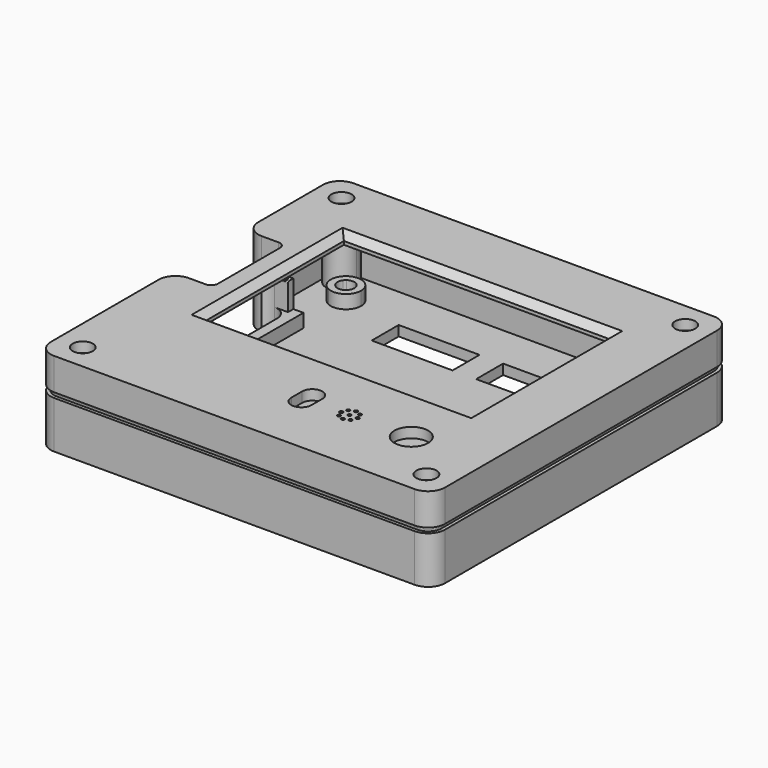
from build123d import *

# Parameters (mm, degrees)
F0_R        = 2.5
F1_DEPTH    = 15
F2_DEPTH    = 7
F0_W        = 24
F0_H        = 10
F3_DEPTH    = 3
F4_R        = 4
F5_DEPTH    = 14
F6_T1_DEPTH = 14
F7_T1_DEPTH = 14
F9_W        = 7
F9_H        = 1
F10_DEPTH   = 8
F9_R        = 0.5
F9_R_2      = 5
F9_W_2      = 79
F9_H_2      = 52
F11_DEPTH   = 3
F12_SIZE    = 2
F13_DEPTH   = 9.5
F14_R       = 0.5
F15_R       = 0.5
F9_R_3      = 1.75
F16_DEPTH   = 8
F17_R       = 3
F18_DEPTH   = 3
F19_R       = 2
F20_W       = 33
F20_H       = 2
F21_DEPTH   = 1


# Not quite as in the source:
# - a fillet or chamfer that OpenCascade refuses, or shapes differently, is made with other operations: its cross-section is extruded or revolved along the edge and cut away or added
# - a feature names something its author has since deleted; it is built from what else it names


with BuildPart() as f1:
    # F0 (on Top) → F1 (new body)
    with BuildSketch(Plane.XY):
        with BuildLine():
            Line((-46.5, 22.5), (-46.5, 24.5))
            Line((-46.5, 24.5), (-50.5, 24.5))
            ThreePointArc((-50.5, 24.5), (-54.0355339059, 25.9644660941), (-55.5, 29.5))
            Line((-55.5, 29.5), (-55.5, 48))
            ThreePointArc((-55.5, 48), (-54.1819805153, 51.1819805153), (-51, 52.5))
            Line((-51, 52.5), (51, 52.5))
            ThreePointArc((51, 52.5), (54.1819805153, 51.1819805153), (55.5, 48))
            Line((55.5, 48), (55.5, -48))
            ThreePointArc((55.5, -48), (54.1819805153, -51.1819805153), (51, -52.5))
            Line((51, -52.5), (-51, -52.5))
            ThreePointArc((-51, -52.5), (-54.1819805153, -51.1819805153), (-55.5, -48))
            Line((-55.5, -48), (-55.5, -13.5))
            ThreePointArc((-55.5, -13.5), (-54.0355339059, -9.9644660941), (-50.5, -8.5))
            Line((-50.5, -8.5), (-46.5, -8.5))
            Line((-46.5, -8.5), (-46.5, -6.5))
            Line((-46.5, -6.5), (-53.5, -6.5))
            ThreePointArc((-53.5, -6.5), (-56.3284271247, -7.6715728753), (-57.5, -10.5))
            Line((-57.5, -10.5), (-57.5, -50.5))
            ThreePointArc((-57.5, -50.5), (-56.3284271247, -53.3284271247), (-53.5, -54.5))
            Line((-53.5, -54.5), (53.5, -54.5))
            ThreePointArc((53.5, -54.5), (56.3284271247, -53.3284271247), (57.5, -50.5))
            Line((57.5, -50.5), (57.5, 50.5))
            ThreePointArc((57.5, 50.5), (56.3284271247, 53.3284271247), (53.5, 54.5))
            Line((53.5, 54.5), (-53.5, 54.5))
            ThreePointArc((-53.5, 54.5), (-56.3284271247, 53.3284271247), (-57.5, 50.5))
            Line((-57.5, 50.5), (-57.5, 26.5))
            ThreePointArc((-57.5, 26.5), (-56.3284271247, 23.6715728753), (-53.5, 22.5))
            Line((-53.5, 22.5), (-46.5, 22.5))
        make_face()
        with BuildLine():
            ThreePointArc((-51, 52.5), (-54.1819805153, 51.1819805153), (-55.5, 48))
            ThreePointArc((-55.5, 48), (-51, 43.5), (-46.5, 48))
            ThreePointArc((-46.5, 48), (-47.8180194847, 51.1819805153), (-51, 52.5))
        make_face()
        with Locations((-51, 48)):
            Circle(F0_R, mode=Mode.SUBTRACT)
        with BuildLine():
            ThreePointArc((55.5, 48), (54.1819805153, 51.1819805153), (51, 52.5))
            ThreePointArc((51, 52.5), (47.8180194847, 44.8180194847), (55.5, 48))
        make_face()
        with Locations((51, 48)):
            Circle(F0_R, mode=Mode.SUBTRACT)
        with BuildLine():
            ThreePointArc((51, -52.5), (54.1819805153, -51.1819805153), (55.5, -48))
            ThreePointArc((55.5, -48), (47.8180194847, -44.8180194847), (51, -52.5))
        make_face()
        with Locations((51, -48)):
            Circle(F0_R, mode=Mode.SUBTRACT)
        with BuildLine():
            ThreePointArc((-46.5, -48), (-51, -43.5), (-55.5, -48))
            ThreePointArc((-55.5, -48), (-54.1819805153, -51.1819805153), (-51, -52.5))
            ThreePointArc((-51, -52.5), (-47.8180194847, -51.1819805153), (-46.5, -48))
        make_face()
        with Locations((-51, -48)):
            Circle(F0_R, mode=Mode.SUBTRACT)
    extrude(amount=F1_DEPTH)

    # F0 (on Top) → F2, piece 5 (join)
    with BuildSketch(Plane.XY):
        Polygon((-43.5, 24.5), (-46.5, 24.5), (-46.5, 22.5), (-46.5, 21.5), (-46.5, -5.5), (-46.5, -6.5), (-46.5, -8.5), (-43.5, -8.5), align=None)
    extrude(amount=F2_DEPTH)



with BuildPart() as f2:
    # F0 (on Top) → F2 (new body)
    with BuildSketch(Plane.XY):
        with BuildLine():
            Line((-46.5, 43), (-46.5, 43.5))
            Line((-46.5, 43.5), (-46, 43.5))
            ThreePointArc((-46, 43.5), (-44.5, 44), (-43, 43.5))
            Line((-43, 43.5), (-40.4688711259, 43.5))
            ThreePointArc((-40.4688711259, 43.5), (-47.6819805153, 44.6819805153), (-46.5, 37.4688711259))
            Line((-46.5, 37.4688711259), (-46.5, 40))
            ThreePointArc((-46.5, 40), (-47, 41.5), (-46.5, 43))
        make_face()
        with BuildLine():
            Line((-40.4688711259, 43.5), (-43, 43.5))
            ThreePointArc((-43, 43.5), (-42.2639320225, 42.6180339887), (-42, 41.5))
            ThreePointArc((-42, 41.5), (-43.709430585, 39.1282917549), (-46.5, 40))
            Line((-46.5, 40), (-46.5, 37.4688711259))
            ThreePointArc((-46.5, 37.4688711259), (-42.1282917549, 37.6757353648), (-40, 41.5))
            ThreePointArc((-40, 41.5), (-40.1187855603, 42.5271124735), (-40.4688711259, 43.5))
        make_face()
        with BuildLine():
            Line((-46, 43.5), (-46.5, 43.5))
            Line((-46.5, 43.5), (-46.5, 43))
            ThreePointArc((-46.5, 43), (-46.267766953, 43.267766953), (-46, 43.5))
        make_face()
    extrude(amount=F2_DEPTH)


with BuildPart() as f2b:
    # F0 (on Top) → F2, piece 2 (new body)
    with BuildSketch(Plane.XY):
        with BuildLine():
            ThreePointArc((49, 41.5), (45.5271124735, 45.8812144397), (40.4688711259, 43.5))
            Line((40.4688711259, 43.5), (43, 43.5))
            ThreePointArc((43, 43.5), (44.5, 44), (46, 43.5))
            Line((46, 43.5), (46.5, 43.5))
            Line((46.5, 43.5), (46.5, 43))
            ThreePointArc((46.5, 43), (46.8717082451, 42.290569415), (47, 41.5))
            ThreePointArc((47, 41.5), (46.8717082451, 40.709430585), (46.5, 40))
            Line((46.5, 40), (46.5, 37.4688711259))
            ThreePointArc((46.5, 37.4688711259), (48.3242646352, 39.1282917549), (49, 41.5))
        make_face()
        with BuildLine():
            Line((43, 43.5), (40.4688711259, 43.5))
            ThreePointArc((40.4688711259, 43.5), (41.3180194847, 38.3180194847), (46.5, 37.4688711259))
            Line((46.5, 37.4688711259), (46.5, 40))
            ThreePointArc((46.5, 40), (42.732233047, 39.732233047), (43, 43.5))
        make_face()
        with BuildLine():
            Line((46.5, 43.5), (46, 43.5))
            ThreePointArc((46, 43.5), (46.267766953, 43.267766953), (46.5, 43))
            Line((46.5, 43), (46.5, 43.5))
        make_face()
    extrude(amount=F2_DEPTH)


with BuildPart() as f2c:
    # F0 (on Top) → F2, piece 3 (new body)
    with BuildSketch(Plane.XY):
        with BuildLine():
            ThreePointArc((-40, -23.5), (-42.1282917549, -19.6757353648), (-46.5, -19.4688711259))
            Line((-46.5, -19.4688711259), (-46.5, -22))
            ThreePointArc((-46.5, -22), (-43.709430585, -21.1282917549), (-42, -23.5))
            ThreePointArc((-42, -23.5), (-43.709430585, -25.8717082451), (-46.5, -25))
            Line((-46.5, -25), (-46.5, -27.5311288741))
            ThreePointArc((-46.5, -27.5311288741), (-42.1282917549, -27.3242646352), (-40, -23.5))
        make_face()
        with BuildLine():
            Line((-46.5, -22), (-46.5, -19.4688711259))
            ThreePointArc((-46.5, -19.4688711259), (-49, -23.5), (-46.5, -27.5311288741))
            Line((-46.5, -27.5311288741), (-46.5, -25))
            ThreePointArc((-46.5, -25), (-47, -23.5), (-46.5, -22))
        make_face()
    extrude(amount=F2_DEPTH)


with BuildPart() as f2d:
    # F0 (on Top) → F2, piece 4 (new body)
    with BuildSketch(Plane.XY):
        with BuildLine():
            Line((46.5, -22), (46.5, -19.4688711259))
            ThreePointArc((46.5, -19.4688711259), (40, -23.5), (46.5, -27.5311288741))
            Line((46.5, -27.5311288741), (46.5, -25))
            ThreePointArc((46.5, -25), (42, -23.5), (46.5, -22))
        make_face()
        with BuildLine():
            ThreePointArc((49, -23.5), (48.3242646352, -21.1282917549), (46.5, -19.4688711259))
            Line((46.5, -19.4688711259), (46.5, -22))
            ThreePointArc((46.5, -22), (46.8717082451, -22.709430585), (47, -23.5))
            ThreePointArc((47, -23.5), (46.8717082451, -24.290569415), (46.5, -25))
            Line((46.5, -25), (46.5, -27.5311288741))
            ThreePointArc((46.5, -27.5311288741), (48.3242646352, -25.8717082451), (49, -23.5))
        make_face()
    extrude(amount=F2_DEPTH)


with BuildPart() as f1_1:
    add(f1.part)

    add(f2.part)  # F3 merges F2

    add(f2b.part)  # F3 merges F2b

    add(f2c.part)  # F3 merges F2c

    add(f2d.part)  # F3 merges F2d
    # F0 (on Top) → F3 (join)
    with BuildSketch(Plane.XY):
        with BuildLine():
            Line((46.5, 43.5), (46, 43.5))
            ThreePointArc((46, 43.5), (46.267766953, 43.267766953), (46.5, 43))
            Line((46.5, 43), (46.5, 43.5))
        make_face()
        with BuildLine():
            ThreePointArc((-46.5, 37.4688711259), (-47.6819805153, 44.6819805153), (-40.4688711259, 43.5))
            Line((-40.4688711259, 43.5), (40.4688711259, 43.5))
            ThreePointArc((40.4688711259, 43.5), (45.5271124735, 45.8812144397), (49, 41.5))
            ThreePointArc((49, 41.5), (48.3242646352, 39.1282917549), (46.5, 37.4688711259))
            Line((46.5, 37.4688711259), (46.5, -19.4688711259))
            ThreePointArc((46.5, -19.4688711259), (48.3242646352, -21.1282917549), (49, -23.5))
            ThreePointArc((49, -23.5), (48.3242646352, -25.8717082451), (46.5, -27.5311288741))
            Line((46.5, -27.5311288741), (46.5, -43.5))
            Line((46.5, -43.5), (-46.5, -43.5))
            Line((-46.5, -43.5), (-46.5, -27.5311288741))
            ThreePointArc((-46.5, -27.5311288741), (-49, -23.5), (-46.5, -19.4688711259))
            Line((-46.5, -19.4688711259), (-46.5, -8.5))
            Line((-46.5, -8.5), (-50.5, -8.5))
            ThreePointArc((-50.5, -8.5), (-54.0355339059, -9.9644660941), (-55.5, -13.5))
            Line((-55.5, -13.5), (-55.5, -48))
            ThreePointArc((-55.5, -48), (-51, -43.5), (-46.5, -48))
            ThreePointArc((-46.5, -48), (-47.8180194847, -51.1819805153), (-51, -52.5))
            Line((-51, -52.5), (51, -52.5))
            ThreePointArc((51, -52.5), (47.8180194847, -44.8180194847), (55.5, -48))
            Line((55.5, -48), (55.5, 48))
            ThreePointArc((55.5, 48), (47.8180194847, 44.8180194847), (51, 52.5))
            Line((51, 52.5), (-51, 52.5))
            ThreePointArc((-51, 52.5), (-47.8180194847, 51.1819805153), (-46.5, 48))
            ThreePointArc((-46.5, 48), (-51, 43.5), (-55.5, 48))
            Line((-55.5, 48), (-55.5, 29.5))
            ThreePointArc((-55.5, 29.5), (-54.0355339059, 25.9644660941), (-50.5, 24.5))
            Line((-50.5, 24.5), (-46.5, 24.5))
            Line((-46.5, 24.5), (-46.5, 37.4688711259))
        make_face()
        with BuildLine():
            Line((40.4688711259, 43.5), (-40.4688711259, 43.5))
            ThreePointArc((-40.4688711259, 43.5), (-40.1187855603, 42.5271124735), (-40, 41.5))
            ThreePointArc((-40, 41.5), (-42.1282917549, 37.6757353648), (-46.5, 37.4688711259))
            Line((-46.5, 37.4688711259), (-46.5, 24.5))
            Line((-46.5, 24.5), (-43.5, 24.5))
            Line((-43.5, 24.5), (-43.5, -8.5))
            Line((-43.5, -8.5), (-46.5, -8.5))
            Line((-46.5, -8.5), (-46.5, -19.4688711259))
            ThreePointArc((-46.5, -19.4688711259), (-42.1282917549, -19.6757353648), (-40, -23.5))
            ThreePointArc((-40, -23.5), (-42.1282917549, -27.3242646352), (-46.5, -27.5311288741))
            Line((-46.5, -27.5311288741), (-46.5, -43.5))
            Line((-46.5, -43.5), (46.5, -43.5))
            Line((46.5, -43.5), (46.5, -27.5311288741))
            ThreePointArc((46.5, -27.5311288741), (40, -23.5), (46.5, -19.4688711259))
            Line((46.5, -19.4688711259), (46.5, 37.4688711259))
            ThreePointArc((46.5, 37.4688711259), (41.3180194847, 38.3180194847), (40.4688711259, 43.5))
        make_face()
        with Locations((-15.25, 34.5)):
            Rectangle(F0_W, F0_H, mode=Mode.SUBTRACT)
        with Locations((15.75, 34.5)):
            Rectangle(F0_W, F0_H, mode=Mode.SUBTRACT)
    extrude(amount=F3_DEPTH)

    # F4
    f4_edges = [f1_1.edges().sort_by_distance(p)[0] for p in [
        (-46.5, 22.5, 3.5),
        (-46.5, -6.5, 3.5),
    ]]
    fillet(f4_edges, radius=F4_R)

    # F0 (on Top) → F5 (join)
    with BuildSketch(Plane.XY):
        with BuildLine():
            Line((-53.5, 21.5), (-53.5, 22.5))
            ThreePointArc((-53.5, 22.5), (-56.3284271247, 23.6715728753), (-57.5, 26.5))
            Line((-57.5, 26.5), (-57.5, 50.5))
            ThreePointArc((-57.5, 50.5), (-56.3284271247, 53.3284271247), (-53.5, 54.5))
            Line((-53.5, 54.5), (53.5, 54.5))
            ThreePointArc((53.5, 54.5), (56.3284271247, 53.3284271247), (57.5, 50.5))
            Line((57.5, 50.5), (57.5, -50.5))
            ThreePointArc((57.5, -50.5), (56.3284271247, -53.3284271247), (53.5, -54.5))
            Line((53.5, -54.5), (-53.5, -54.5))
            ThreePointArc((-53.5, -54.5), (-56.3284271247, -53.3284271247), (-57.5, -50.5))
            Line((-57.5, -50.5), (-57.5, -10.5))
            ThreePointArc((-57.5, -10.5), (-56.3284271247, -7.6715728753), (-53.5, -6.5))
            Line((-53.5, -6.5), (-53.5, -5.5))
            ThreePointArc((-53.5, -5.5), (-57.0355339059, -6.9644660941), (-58.5, -10.5))
            Line((-58.5, -10.5), (-58.5, -50.5))
            ThreePointArc((-58.5, -50.5), (-57.0355339059, -54.0355339059), (-53.5, -55.5))
            Line((-53.5, -55.5), (53.5, -55.5))
            ThreePointArc((53.5, -55.5), (57.0355339059, -54.0355339059), (58.5, -50.5))
            Line((58.5, -50.5), (58.5, 50.5))
            ThreePointArc((58.5, 50.5), (57.0355339059, 54.0355339059), (53.5, 55.5))
            Line((53.5, 55.5), (-53.5, 55.5))
            ThreePointArc((-53.5, 55.5), (-57.0355339059, 54.0355339059), (-58.5, 50.5))
            Line((-58.5, 50.5), (-58.5, 26.5))
            ThreePointArc((-58.5, 26.5), (-57.0355339059, 22.9644660941), (-53.5, 21.5))
        make_face()
    extrude(amount=F5_DEPTH)

    # F6: fillet of radius 5 on 2 edges, made by hand

    # F6_s2 → F6_t1 (join)
    with BuildSketch(Plane.XY):
        with BuildLine():
            ThreePointArc((-50.5, 22.5), (-52.0811388301, 22.2434164903), (-53.5, 21.5))
            Line((-53.5, 21.5), (-53.5, 22.5))
            Line((-53.5, 22.5), (-50.5, 22.5))
        make_face()
    extrude(amount=F6_T1_DEPTH)

    # F7: fillet of radius 5 on 2 edges, made by hand

    # F7_s2 → F7_t1 (join)
    with BuildSketch(Plane.XY):
        with BuildLine():
            ThreePointArc((-50.5, -6.5), (-52.0811388301, -6.2434164903), (-53.5, -5.5))
            Line((-53.5, -5.5), (-53.5, -6.5))
            Line((-53.5, -6.5), (-50.5, -6.5))
        make_face()
    extrude(amount=F7_T1_DEPTH)

    # F15
    f15_edges = [f1_1.edges().sort_by_distance(p)[0] for p in [
        (0, 54.5, 15),
        (-50, -6.5, 15),
        (-50, 22.5, 15),
        (-56.328427, -7.671573, 15),
        (-56.328427, 23.671573, 15),
        (-57.5, -30.5, 15),
        (-56.328427, -53.328427, 15),
        (0, -54.5, 15),
        (56.328427, -53.328427, 15),
        (57.5, 0, 15),
        (56.328427, 53.328427, 15),
        (-56.328427, 53.328427, 15),
        (-57.5, 38.5, 15),
    ]]
    fillet(f15_edges, radius=F15_R)


with BuildPart() as f10:
    # F9 (on offset) → F10 (new body)
    with BuildSketch(Plane.XY.offset(25)):
        with BuildLine():
            Line((-53.5, 21.5), (-53.5, 22.5))
            ThreePointArc((-53.5, 22.5), (-56.3284271247, 23.6715728753), (-57.5, 26.5))
            Line((-57.5, 26.5), (-57.5, 50.5))
            ThreePointArc((-57.5, 50.5), (-56.3284271247, 53.3284271247), (-53.5, 54.5))
            Line((-53.5, 54.5), (53.5, 54.5))
            ThreePointArc((53.5, 54.5), (56.3284271247, 53.3284271247), (57.5, 50.5))
            Line((57.5, 50.5), (57.5, -50.5))
            ThreePointArc((57.5, -50.5), (56.3284271247, -53.3284271247), (53.5, -54.5))
            Line((53.5, -54.5), (-53.5, -54.5))
            ThreePointArc((-53.5, -54.5), (-56.3284271247, -53.3284271247), (-57.5, -50.5))
            Line((-57.5, -50.5), (-57.5, -10.5))
            ThreePointArc((-57.5, -10.5), (-56.3284271247, -7.6715728753), (-53.5, -6.5))
            Line((-53.5, -6.5), (-53.5, -5.5))
            ThreePointArc((-53.5, -5.5), (-57.0355339059, -6.9644660941), (-58.5, -10.5))
            Line((-58.5, -10.5), (-58.5, -50.5))
            ThreePointArc((-58.5, -50.5), (-57.0355339059, -54.0355339059), (-53.5, -55.5))
            Line((-53.5, -55.5), (53.5, -55.5))
            ThreePointArc((53.5, -55.5), (57.0355339059, -54.0355339059), (58.5, -50.5))
            Line((58.5, -50.5), (58.5, 50.5))
            ThreePointArc((58.5, 50.5), (57.0355339059, 54.0355339059), (53.5, 55.5))
            Line((53.5, 55.5), (-53.5, 55.5))
            ThreePointArc((-53.5, 55.5), (-57.0355339059, 54.0355339059), (-58.5, 50.5))
            Line((-58.5, 50.5), (-58.5, 26.5))
            ThreePointArc((-58.5, 26.5), (-57.0355339059, 22.9644660941), (-53.5, 21.5))
        make_face()
        with Locations((-50, 22)):
            Rectangle(F9_W, F9_H)
        with BuildLine():
            Line((-46.5, 22.5), (-46.5, 24.5))
            Line((-46.5, 24.5), (-50.5, 24.5))
            ThreePointArc((-50.5, 24.5), (-54.0355339059, 25.9644660941), (-55.5, 29.5))
            Line((-55.5, 29.5), (-55.5, 48))
            ThreePointArc((-55.5, 48), (-54.1819805153, 51.1819805153), (-51, 52.5))
            Line((-51, 52.5), (51, 52.5))
            ThreePointArc((51, 52.5), (54.1819805153, 51.1819805153), (55.5, 48))
            Line((55.5, 48), (55.5, -48))
            ThreePointArc((55.5, -48), (54.1819805153, -51.1819805153), (51, -52.5))
            Line((51, -52.5), (-51, -52.5))
            ThreePointArc((-51, -52.5), (-54.1819805153, -51.1819805153), (-55.5, -48))
            Line((-55.5, -48), (-55.5, -13.5))
            ThreePointArc((-55.5, -13.5), (-54.0355339059, -9.9644660941), (-50.5, -8.5))
            Line((-50.5, -8.5), (-46.5, -8.5))
            Line((-46.5, -8.5), (-46.5, -6.5))
            Line((-46.5, -6.5), (-53.5, -6.5))
            ThreePointArc((-53.5, -6.5), (-56.3284271247, -7.6715728753), (-57.5, -10.5))
            Line((-57.5, -10.5), (-57.5, -50.5))
            ThreePointArc((-57.5, -50.5), (-56.3284271247, -53.3284271247), (-53.5, -54.5))
            Line((-53.5, -54.5), (53.5, -54.5))
            ThreePointArc((53.5, -54.5), (56.3284271247, -53.3284271247), (57.5, -50.5))
            Line((57.5, -50.5), (57.5, 50.5))
            ThreePointArc((57.5, 50.5), (56.3284271247, 53.3284271247), (53.5, 54.5))
            Line((53.5, 54.5), (-53.5, 54.5))
            ThreePointArc((-53.5, 54.5), (-56.3284271247, 53.3284271247), (-57.5, 50.5))
            Line((-57.5, 50.5), (-57.5, 26.5))
            ThreePointArc((-57.5, 26.5), (-56.3284271247, 23.6715728753), (-53.5, 22.5))
            Line((-53.5, 22.5), (-46.5, 22.5))
        make_face()
        with Locations((-50, -6)):
            Rectangle(F9_W, F9_H)
    extrude(amount=-F10_DEPTH)

    # F9 (on offset) → F11 (join)
    with BuildSketch(Plane.XY.offset(25)):
        with BuildLine():
            Line((-46.5, 24.5), (-46.5, 43.5))
            Line((-46.5, 43.5), (46.5, 43.5))
            Line((46.5, 43.5), (46.5, -43.5))
            Line((46.5, -43.5), (-46.5, -43.5))
            Line((-46.5, -43.5), (-46.5, -8.5))
            Line((-46.5, -8.5), (-50.5, -8.5))
            ThreePointArc((-50.5, -8.5), (-54.0355339059, -9.9644660941), (-55.5, -13.5))
            Line((-55.5, -13.5), (-55.5, -48))
            ThreePointArc((-55.5, -48), (-51, -43.5), (-46.5, -48))
            ThreePointArc((-46.5, -48), (-47.8180194847, -51.1819805153), (-51, -52.5))
            Line((-51, -52.5), (51, -52.5))
            ThreePointArc((51, -52.5), (47.8180194847, -44.8180194847), (55.5, -48))
            Line((55.5, -48), (55.5, 48))
            ThreePointArc((55.5, 48), (47.8180194847, 44.8180194847), (51, 52.5))
            Line((51, 52.5), (-51, 52.5))
            ThreePointArc((-51, 52.5), (-47.8180194847, 51.1819805153), (-46.5, 48))
            ThreePointArc((-46.5, 48), (-51, 43.5), (-55.5, 48))
            Line((-55.5, 48), (-55.5, 29.5))
            ThreePointArc((-55.5, 29.5), (-54.0355339059, 25.9644660941), (-50.5, 24.5))
            Line((-50.5, 24.5), (-46.5, 24.5))
        make_face()
        Polygon((46.5, 43.5), (-46.5, 43.5), (-46.5, 24.5), (-45.5, 24.5), (-45.5, -8.5), (-46.5, -8.5), (-46.5, -43.5), (46.5, -43.5), align=None)
        with BuildLine():
            ThreePointArc((2.5, -33.5), (5.5, -30.5), (8.5, -33.5))
            Line((8.5, -33.5), (8.5, -37.5))
            ThreePointArc((8.5, -37.5), (5.5, -40.5), (2.5, -37.5))
            Line((2.5, -37.5), (2.5, -33.5))
        make_face(mode=Mode.SUBTRACT)
        with Locations((18.5, -38.3816510439)):
            Circle(F9_R, mode=Mode.SUBTRACT)
        with Locations((16.7735965964, -37.66655134)):
            Circle(F9_R, mode=Mode.SUBTRACT)
        with Locations((16.0584968925, -35.9401479363)):
            Circle(F9_R, mode=Mode.SUBTRACT)
        with Locations((20.2264034036, -37.66655134)):
            Circle(F9_R, mode=Mode.SUBTRACT)
        with Locations((18.5, -35.9401479363)):
            Circle(F9_R, mode=Mode.SUBTRACT)
        with Locations((20.9415031075, -35.9401479363)):
            Circle(F9_R, mode=Mode.SUBTRACT)
        with Locations((16.7735965964, -34.2137445327)):
            Circle(F9_R, mode=Mode.SUBTRACT)
        with Locations((18.5, -33.4986448288)):
            Circle(F9_R, mode=Mode.SUBTRACT)
        with Locations((20.2264034036, -34.2137445327)):
            Circle(F9_R, mode=Mode.SUBTRACT)
        with Locations((36.5, -35.5)):
            Circle(F9_R_2, mode=Mode.SUBTRACT)
        with Locations((0, 8.5)):
            Rectangle(F9_W_2, F9_H_2, mode=Mode.SUBTRACT)
    extrude(amount=-F11_DEPTH)

    # F12
    f12_edges = [f10.edges().sort_by_distance(p)[0] for p in [
        (0, 34.5, 25),
        (-39.5, 8.5, 25),
        (0, -17.5, 25),
        (39.5, 8.5, 25),
    ]]
    chamfer(f12_edges, length=F12_SIZE)

    # F9 (on offset) → F13 (join)
    with BuildSketch(Plane.XY.offset(25)):
        with BuildLine():
            Line((-53.5, 21.5), (-53.5, 22.5))
            ThreePointArc((-53.5, 22.5), (-56.3284271247, 23.6715728753), (-57.5, 26.5))
            Line((-57.5, 26.5), (-57.5, 50.5))
            ThreePointArc((-57.5, 50.5), (-56.3284271247, 53.3284271247), (-53.5, 54.5))
            Line((-53.5, 54.5), (53.5, 54.5))
            ThreePointArc((53.5, 54.5), (56.3284271247, 53.3284271247), (57.5, 50.5))
            Line((57.5, 50.5), (57.5, -50.5))
            ThreePointArc((57.5, -50.5), (56.3284271247, -53.3284271247), (53.5, -54.5))
            Line((53.5, -54.5), (-53.5, -54.5))
            ThreePointArc((-53.5, -54.5), (-56.3284271247, -53.3284271247), (-57.5, -50.5))
            Line((-57.5, -50.5), (-57.5, -10.5))
            ThreePointArc((-57.5, -10.5), (-56.3284271247, -7.6715728753), (-53.5, -6.5))
            Line((-53.5, -6.5), (-53.5, -5.5))
            ThreePointArc((-53.5, -5.5), (-57.0355339059, -6.9644660941), (-58.5, -10.5))
            Line((-58.5, -10.5), (-58.5, -50.5))
            ThreePointArc((-58.5, -50.5), (-57.0355339059, -54.0355339059), (-53.5, -55.5))
            Line((-53.5, -55.5), (53.5, -55.5))
            ThreePointArc((53.5, -55.5), (57.0355339059, -54.0355339059), (58.5, -50.5))
            Line((58.5, -50.5), (58.5, 50.5))
            ThreePointArc((58.5, 50.5), (57.0355339059, 54.0355339059), (53.5, 55.5))
            Line((53.5, 55.5), (-53.5, 55.5))
            ThreePointArc((-53.5, 55.5), (-57.0355339059, 54.0355339059), (-58.5, 50.5))
            Line((-58.5, 50.5), (-58.5, 26.5))
            ThreePointArc((-58.5, 26.5), (-57.0355339059, 22.9644660941), (-53.5, 21.5))
        make_face()
        with Locations((-50, -6)):
            Rectangle(F9_W, F9_H)
        with Locations((-50, 22)):
            Rectangle(F9_W, F9_H)
    extrude(amount=-F13_DEPTH)

    # F14
    f14_edges = [f10.edges().sort_by_distance(p)[0] for p in [
        (-57.5, 38.5, 15.5),
    ]]
    fillet(f14_edges, radius=F14_R)

    # F9 (on offset) → F16 (join)
    with BuildSketch(Plane.XY.offset(25)):
        with BuildLine():
            ThreePointArc((55.5, 48), (54.1819805153, 51.1819805153), (51, 52.5))
            ThreePointArc((51, 52.5), (47.8180194847, 44.8180194847), (55.5, 48))
        make_face()
        with Locations((51, 48)):
            Circle(F9_R_3, mode=Mode.SUBTRACT)
        with BuildLine():
            ThreePointArc((-51, 52.5), (-54.1819805153, 51.1819805153), (-55.5, 48))
            ThreePointArc((-55.5, 48), (-51, 43.5), (-46.5, 48))
            ThreePointArc((-46.5, 48), (-47.8180194847, 51.1819805153), (-51, 52.5))
        make_face()
        with Locations((-51, 48)):
            Circle(F9_R_3, mode=Mode.SUBTRACT)
        with BuildLine():
            ThreePointArc((51, -52.5), (54.1819805153, -51.1819805153), (55.5, -48))
            ThreePointArc((55.5, -48), (47.8180194847, -44.8180194847), (51, -52.5))
        make_face()
        with Locations((51, -48)):
            Circle(F9_R_3, mode=Mode.SUBTRACT)
        with BuildLine():
            ThreePointArc((-46.5, -48), (-51, -43.5), (-55.5, -48))
            ThreePointArc((-55.5, -48), (-54.1819805153, -51.1819805153), (-51, -52.5))
            ThreePointArc((-51, -52.5), (-47.8180194847, -51.1819805153), (-46.5, -48))
        make_face()
        with Locations((-51, -48)):
            Circle(F9_R_3, mode=Mode.SUBTRACT)
        Polygon((-45.5, 24.5), (-46.5, 24.5), (-46.5, 22.5), (-46.5, 21.5), (-46.5, -5.5), (-46.5, -6.5), (-46.5, -8.5), (-45.5, -8.5), align=None)
    extrude(amount=-F16_DEPTH)

    # F17 (on face) → F18 (cut)
    with BuildSketch(Plane.XY.offset(25)):
        with Locations((51, 48)):
            Circle(F17_R)
        with Locations((-51, 48)):
            Circle(F17_R)
        with Locations((-51, -48)):
            Circle(F17_R)
        with Locations((51, -48)):
            Circle(F17_R)
    extrude(amount=-F18_DEPTH, mode=Mode.SUBTRACT)

    # F19
    f19_edges = [f10.edges().sort_by_distance(p)[0] for p in [
        (-46.5, 21.5, 21),
        (-46.5, -5.5, 21),
    ]]
    fillet(f19_edges, radius=F19_R)

    # F20 (on face) → F21 (cut)
    with BuildSketch(Plane.YZ.offset(-45.5)):
        with Locations((8, 18)):
            Rectangle(F20_W, F20_H)
    extrude(amount=-F21_DEPTH, mode=Mode.SUBTRACT)


solid = Compound([f1_1.part, f10.part])
